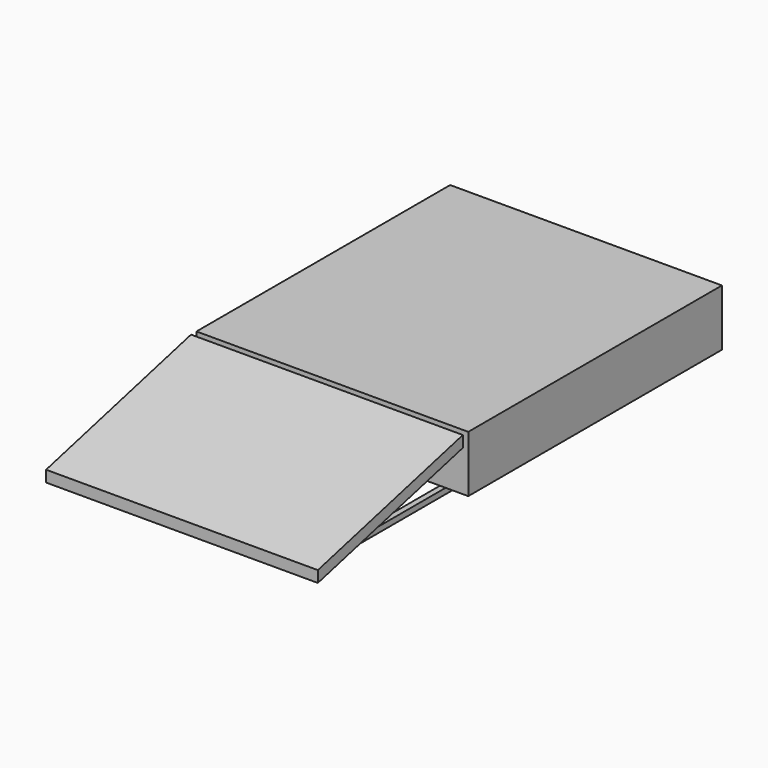
from build123d import *

# Parameters (mm, degrees)
F0_W       = 95
F0_H       = 2.5
F0_W_2     = 2.5
F0_H_2     = 22
F0_H_3     = 3
F1_DEPTH   = 2.5
F0_H_4     = 99.75
F0_H_5     = 13.25
F2_DEPTH   = 25
F0_H_6     = 61
F3_DEPTH   = 25
F4_SIZE2   = 19.99999
F4_SIZE    = 79.99999
F4_2_SIZE2 = 19.99999
F4_2_SIZE  = 79.99999


# Not quite as in the source:
# - a fillet or chamfer is up to 0.001 mm smaller than in the source, because OpenCascade refuses the exact size


with BuildPart() as f1:
    # F0 (on Top) → F1 (new body)
    with BuildSketch(Plane.XY):
        Polygon((-47.5, 118), (-50, 118), (-50, 0), (-47.5, 0), (-47.5, 2.5), (-47.5, 102.25), (-47.5, 104.75), align=None)
        Polygon((50, 121.5), (-50, 121.5), (-50, 118), (-47.5, 118), (-47.5, 119), (47.5, 119), (47.5, 118), (50, 118), align=None)
        with Locations((0, 103.5)):
            Rectangle(F0_W, F0_H)
        Polygon((50, 0), (50, 118), (47.5, 118), (47.5, 104.75), (47.5, 102.25), (47.5, 2.5), (47.5, 0), align=None)
        with Locations((0, 1.25)):
            Rectangle(F0_W, F0_H)
        with Locations((-48.75, -11)):
            Rectangle(F0_W_2, F0_H_2)
        Polygon((-47.5, -25), (-50, -25), (-50, -88.5), (50, -88.5), (50, -25), (47.5, -25), (47.5, -86), (-47.5, -86), align=None)
        with Locations((48.75, -11)):
            Rectangle(F0_W_2, F0_H_2)
        with Locations((-48.75, -23.5)):
            Rectangle(F0_W_2, F0_H_3)
        with Locations((48.75, -23.5)):
            Rectangle(F0_W_2, F0_H_3)
    extrude(amount=-F1_DEPTH)


with BuildPart() as f2:
    # F0 (on Top) → F2 (new body)
    with BuildSketch(Plane.XY):
        with Locations((-48.75, -11)):
            Rectangle(F0_W_2, F0_H_2)
        with Locations((0, -11)):
            Rectangle(F0_W, F0_H_2)
        with Locations((48.75, -11)):
            Rectangle(F0_W_2, F0_H_2)
        Polygon((60, 118), (50, 118), (50, 0), (50, -22), (60, -22), align=None)
        with Locations((0, 1.25)):
            Rectangle(F0_W, F0_H)
        Polygon((50, 0), (50, 118), (47.5, 118), (47.5, 104.75), (47.5, 102.25), (47.5, 2.5), (47.5, 0), align=None)
        Polygon((-47.5, 118), (-50, 118), (-50, 0), (-47.5, 0), (-47.5, 2.5), (-47.5, 102.25), (-47.5, 104.75), align=None)
        with Locations((0, 103.5)):
            Rectangle(F0_W, F0_H)
        Polygon((-50, 0), (-50, 118), (-60, 118), (-60, -22), (-50, -22), align=None)
        with Locations((0, 52.375)):
            Rectangle(F0_W, F0_H_4)
        with Locations((0, 111.375)):
            Rectangle(F0_W, F0_H_5)
    extrude(amount=F2_DEPTH)


with BuildPart() as f3:
    # F0 (on Top) → F3 (new body)
    with BuildSketch(Plane.XY):
        Polygon((-50, -88.5), (-50, -25), (-60, -25), (-60, -105), (60, -105), (60, -25), (50, -25), (50, -88.5), align=None)
        Polygon((-47.5, -25), (-50, -25), (-50, -88.5), (50, -88.5), (50, -25), (47.5, -25), (47.5, -86), (-47.5, -86), align=None)
        with Locations((0, -55.5)):
            Rectangle(F0_W, F0_H_6)
    extrude(amount=F3_DEPTH)

    # F4 (size 80 and 20 in the source; OpenCascade refuses exactly that, so slightly less here)
    f4_edges = [f3.edges().sort_by_distance(p)[0] for p in [
        (0, -105, 25),
    ]]
    f4_side = f3.faces().sort_by_distance((0, -65, 25))[0]
    chamfer(f4_edges, length=F4_SIZE, length2=F4_SIZE2, reference=f4_side)

    # F4#2 (size 80 and 20 in the source; OpenCascade refuses exactly that, so slightly less here)
    f4_2_edges = [f3.edges().sort_by_distance(p)[0] for p in [
        (0, -25, 0),
    ]]
    f4_2_side = f3.faces().sort_by_distance((0, -65, 0))[0]
    chamfer(f4_2_edges, length=F4_2_SIZE, length2=F4_2_SIZE2, reference=f4_2_side)


solid = Compound([f1.part, f2.part, f3.part])
